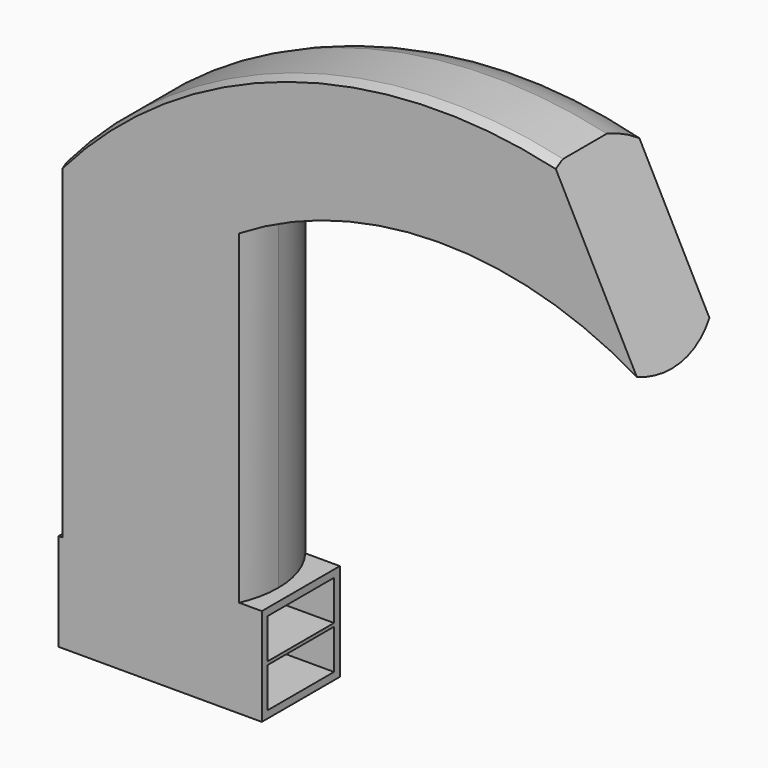
from build123d import *

# Parameters (mm, degrees)
F0_W     = 50
F0_H     = 24
F1_DEPTH = 24
F3_W     = 20.4
F3_H     = 9.8
F4_DEPTH = 50.001
F5_DEPTH = 80
F7_ANGLE = 62.6704880326


with BuildPart() as f1:
    # F0 (on Front) → F1 (new body)
    with BuildSketch(Plane.XZ):
        with Locations((-68.9176678658, 12)):
            Rectangle(F0_W, F0_H)
    extrude(amount=F1_DEPTH)

    # F3 (on face) → F4 (cut, through all)
    with BuildSketch(Plane(origin=(-93.9176678658, 0, 0), x_dir=(0, -1, 0), z_dir=(-1, 0, 0))):
        with Locations((12, 6.7)):
            Rectangle(F3_W, F3_H)
        with Locations((12, 17.3)):
            Rectangle(F3_W, F3_H)
    extrude(amount=-F4_DEPTH, mode=Mode.SUBTRACT)

    # F2 (on face) → F5 (join)
    with BuildSketch(Plane.XY.offset(24)):
        with BuildLine():
            ThreePointArc((-49.4927692396, -24), (-47.9986026074, -19.3399762696), (-47.4933667129, -14.4724212587))
            ThreePointArc((-47.4933667129, -14.4724212587), (-48.7602054242, -6.8275726586), (-52.425289602, 0))
            Line((-52.425289602, 0), (-89.9617876104, 0))
            ThreePointArc((-89.9617876104, 0), (-92.2976878441, -3.6875692563), (-93.9176678658, -7.7409951716))
            Line((-93.9176678658, -7.7409951716), (-93.9176678658, -21.2038473458))
            ThreePointArc((-93.9176678658, -21.2038473458), (-93.4499426711, -22.6180106094), (-92.8943079727, -24))
            Line((-92.8943079727, -24), (-49.4927692396, -24))
        make_face()
    extrude(amount=F5_DEPTH)

    # F6 (on face) → F7 (revolve)
    with BuildSketch(Plane.XY.offset(104)):
        with BuildLine():
            ThreePointArc((-49.4927692396, -24), (-47.9986026074, -19.3399762696), (-47.4933667129, -14.4724212587))
            ThreePointArc((-47.4933667129, -14.4724212587), (-48.7602054242, -6.8275726586), (-52.425289602, 0))
            Line((-52.425289602, 0), (-89.9617876104, 0))
            ThreePointArc((-89.9617876104, 0), (-92.2976878441, -3.6875692563), (-93.9176678658, -7.7409951716))
            Line((-93.9176678658, -7.7409951716), (-93.9176678658, -21.2038473458))
            ThreePointArc((-93.9176678658, -21.2038473458), (-93.4499426711, -22.6180106094), (-92.8943079727, -24))
            Line((-92.8943079727, -24), (-49.4927692396, -24))
        make_face()
    revolve(axis=Axis((0, 2.9759369791, 24), (0, 1, 0)), revolution_arc=F7_ANGLE)


solid = f1.part
